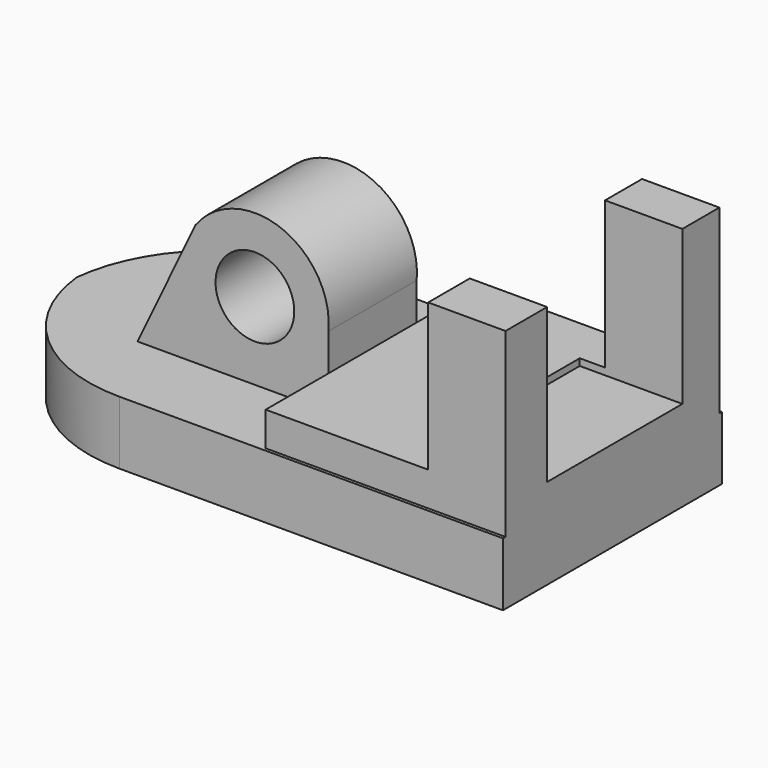
from build123d import *

# Parameters (mm, degrees)
F1_DEPTH    = 54.864
F0_R        = 15.7777597409
F2_DEPTH    = 22.098
F3_DEPTH    = 53.594
F4_T1_DEPTH = 332.0051224214
F5_DEPTH    = 131.826
F6_W        = 67.7949339151
F6_H        = 61.7567202186
F7_DEPTH    = 41.148


# Not quite as in the source:
# - a fillet or chamfer that OpenCascade refuses, or shapes differently, is made with other operations: its cross-section is extruded or revolved along the edge and cut away or added


with BuildPart() as f1:
    # F0 (on Front) → F1 (new body, symmetric)
    with BuildSketch(Plane.XZ):
        Polygon((-107.4633456931, 25.4), (-107.4633456931, 0), (107.6379133128, 0), (107.6379133128, 25.4), (11.4811650322, 25.4), (-65.0678679326, 25.4), align=None)
    extrude(amount=F1_DEPTH, both=True)

    # F0 (on Front) → F2 (join, symmetric)
    with BuildSketch(Plane.XZ):
        with BuildLine():
            Line((-46.6904140055, 63.9219704105), (-65.0678679326, 25.4))
            Line((-65.0678679326, 25.4), (11.4811650322, 25.4))
            Line((11.4811650322, 25.4), (11.4811650322, 39.0391899168))
            Line((11.4811650322, 39.0391899168), (11.4811650322, 53.899857424))
            ThreePointArc((11.4811650322, 53.899857424), (-7.5633921192, 84.1691084188), (-41.8619237654, 74.0432287141))
            Line((-41.8619237654, 74.0432287141), (-46.6904140055, 63.9219704105))
        make_face()
        with Locations((-18.0268805863, 56.4600032051)):
            Circle(F0_R, mode=Mode.SUBTRACT)
    extrude(amount=F2_DEPTH, both=True)

    # F0 (on Front) → F3 (join, symmetric)
    with BuildSketch(Plane.XZ):
        Polygon((11.4811650322, 25.4), (107.6379133128, 25.4), (107.6379133128, 98.0671415215), (76.6363167746, 98.0671415215), (76.6363167746, 39.0391899168), (11.4811650322, 39.0391899168), align=None)
    extrude(amount=F3_DEPTH, both=True)

    # F4: fillet of radius 61.3210244843 on 2 edges, made by hand

    # F4_s2 → F4_t1 (cut)
    with BuildSketch(Plane.XY.offset(-153.3025612107)):
        with BuildLine():
            ThreePointArc((-107.4633456931, -6.4570244843), (-89.502833451, 36.9034877579), (-46.1423212089, 54.864))
            Line((-46.1423212089, 54.864), (-107.4633456931, 54.864))
            Line((-107.4633456931, 54.864), (-107.4633456931, -6.4570244843))
        make_face()
        with BuildLine():
            ThreePointArc((-107.4633456931, 6.4570244843), (-89.502833451, -36.9034877579), (-46.1423212089, -54.864))
            Line((-46.1423212089, -54.864), (-107.4633456931, -54.864))
            Line((-107.4633456931, -54.864), (-107.4633456931, 6.4570244843))
        make_face()
    extrude(amount=F4_T1_DEPTH, mode=Mode.SUBTRACT)

    # F0 (on Front) → F5 (cut)
    with BuildSketch(Plane.XZ):
        with Locations((-18.0268805863, 56.4600032051)):
            Circle(F0_R)
    extrude(amount=-F5_DEPTH, mode=Mode.SUBTRACT)

    # F6 (on face) → F7 (cut)
    with BuildSketch(Plane.YZ.offset(107.6379133128)):
        with Locations((1.151856035, 67.1887814122)):
            Rectangle(F6_W, F6_H)
    extrude(amount=-F7_DEPTH, mode=Mode.SUBTRACT)


solid = f1.part
